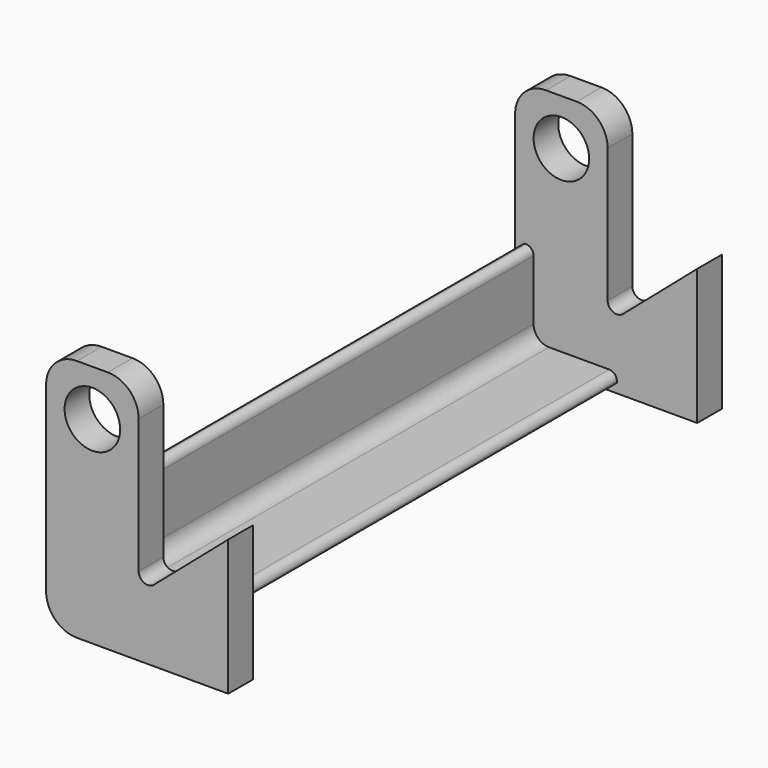
from build123d import *

# Parameters (mm, degrees)
F0_R     = 9
F1_DEPTH = 10
F7_DEPTH = 180
F8_R     = 9
F9_DEPTH = 10


# Not quite as in the source:
# - a feature of the source that left no trace in its solid (it failed there, or was rolled back) is left out


with BuildPart() as f1:
    # F0 (on Front) → F1 (new body)
    with BuildSketch(Plane.XZ):
        with BuildLine():
            Line((5, 15), (-5, 15))
            ThreePointArc((-5, 15), (-12.0710678119, 12.0710678119), (-15, 5))
            Line((-15, 5), (-15, -54))
            ThreePointArc((-15, -54), (-12.0710678119, -61.0710678119), (-5, -64))
            Line((-5, -64), (44.0328441188, -64))
            Line((44.0328441188, -64), (44.0328441188, -20))
            Line((44.0328441188, -20), (19.9575467156, -40.731087613))
            ThreePointArc((19.9575467156, -40.731087613), (16.7495281184, -41.1847233597), (15, -38.4577616671))
            Line((15, -38.4577616671), (15, 5))
            ThreePointArc((15, 5), (12.0710678119, 12.0710678119), (5, 15))
        make_face()
        Circle(F0_R, mode=Mode.SUBTRACT)
    extrude(amount=F1_DEPTH)

    # F6 (on face) → F7 (join)
    with BuildSketch(Plane.XZ.offset(10)):
        with BuildLine():
            Line((-12, -61), (18, -61))
            Line((18, -61), (18, -60.5))
            ThreePointArc((18, -60.5), (17.267766953, -58.732233047), (15.5, -58))
            Line((15.5, -58), (-4, -58))
            ThreePointArc((-4, -58), (-7.5355339059, -56.5355339059), (-9, -53))
            Line((-9, -53), (-9, -33.5))
            ThreePointArc((-9, -33.5), (-9.732233047, -31.732233047), (-11.5, -31))
            Line((-11.5, -31), (-12, -31))
            Line((-12, -31), (-12, -61))
        make_face()
    extrude(amount=F7_DEPTH)

    # F8 (on face) → F9 (join)
    with BuildSketch(Plane.XZ.offset(190)):
        with BuildLine():
            Line((5, 15), (-5, 15))
            ThreePointArc((-5, 15), (-12.0710678119, 12.0710678119), (-15, 5))
            Line((-15, 5), (-15, -54))
            ThreePointArc((-15, -54), (-12.0710678119, -61.0710678119), (-5, -64))
            Line((-5, -64), (44.0328441188, -64))
            Line((44.0328441188, -64), (44.0328441188, -20))
            Line((44.0328441188, -20), (19.9575467156, -40.731087613))
            ThreePointArc((19.9575467156, -40.731087613), (16.7495281184, -41.1847233597), (15, -38.4577616671))
            Line((15, -38.4577616671), (15, 5))
            ThreePointArc((15, 5), (12.0710678119, 12.0710678119), (5, 15))
        make_face()
        Circle(F8_R, mode=Mode.SUBTRACT)
    extrude(amount=F9_DEPTH)


solid = f1.part
